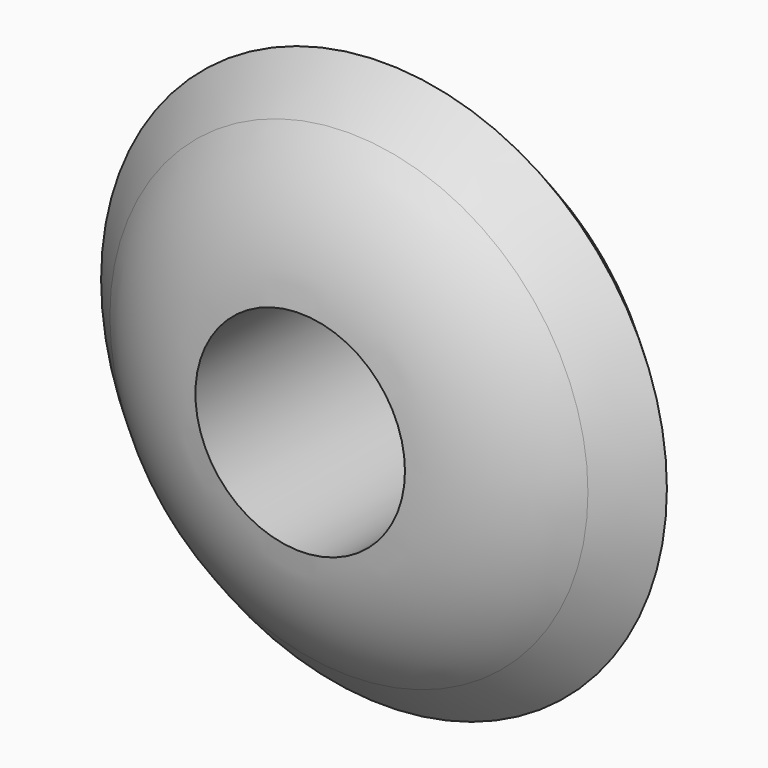
from build123d import *

# Parameters (mm, degrees)
F0_R     = 6.75
F0_R_2   = 2.5
F1_DEPTH = 5
F2_SIZE  = 2.49999


# Not quite as in the source:
# - a fillet or chamfer that OpenCascade refuses, or shapes differently, is made with other operations: its cross-section is extruded or revolved along the edge and cut away or added
# - a fillet or chamfer is up to 0.001 mm smaller than in the source, because OpenCascade refuses the exact size


with BuildPart() as f1:
    # F0 (on Front) → F1 (new body)
    with BuildSketch(Plane.XZ):
        Circle(F0_R)
        Circle(F0_R_2, mode=Mode.SUBTRACT)
    extrude(amount=F1_DEPTH)

    # F2 (size 2.5 in the source; OpenCascade refuses exactly that, so slightly less here)
    f2_edges = [f1.edges().sort_by_distance(p)[0] for p in [
        (-6.75, 0, 0),
        (-6.75, -5, 0),
    ]]
    chamfer(f2_edges, length=F2_SIZE)

    # F3: fillet of radius 5 on 2 edges, made by hand

    # F3_s1 → F3_t2 (revolve, cut)
    with BuildSketch(Plane.XY):
        with BuildLine():
            ThreePointArc((5.7034349304, -3.5465750696), (4.2337560614, -4.5643084484), (2.5, -5))
            Line((2.5, -5), (2.5066419795, -5.0997791767))
            ThreePointArc((2.5066419795, -5.0997791767), (3.375005, -5.1), (4.25001, -5.1))
            Line((4.25001, -5.1), (4.3207206781, -5.0707106781))
            Line((4.3207206781, -5.0707106781), (5.7741456085, -3.6172857477))
            Line((5.7741456085, -3.6172857477), (5.7034349304, -3.5465750696))
        make_face()
    revolve(axis=Axis((0, -5, 0), (0, -1, 0)), mode=Mode.SUBTRACT)

    # F3_s3 → F3_t4 (revolve, cut)
    with BuildSketch(Plane.XY):
        with BuildLine():
            ThreePointArc((5.7034349304, -1.4534249304), (4.2337560614, -0.4356915516), (2.5, 0))
            Line((2.5, 0), (2.5066419795, 0.0997791767))
            ThreePointArc((2.5066419795, 0.0997791767), (3.375005, 0.1), (4.25001, 0.1))
            Line((4.25001, 0.1), (4.3207206781, 0.0707106781))
            Line((4.3207206781, 0.0707106781), (5.7741456085, -1.3827142523))
            Line((5.7741456085, -1.3827142523), (5.7034349304, -1.4534249304))
        make_face()
    revolve(axis=Axis((0, 0, 0), (0, -1, 0)), mode=Mode.SUBTRACT)


solid = f1.part
